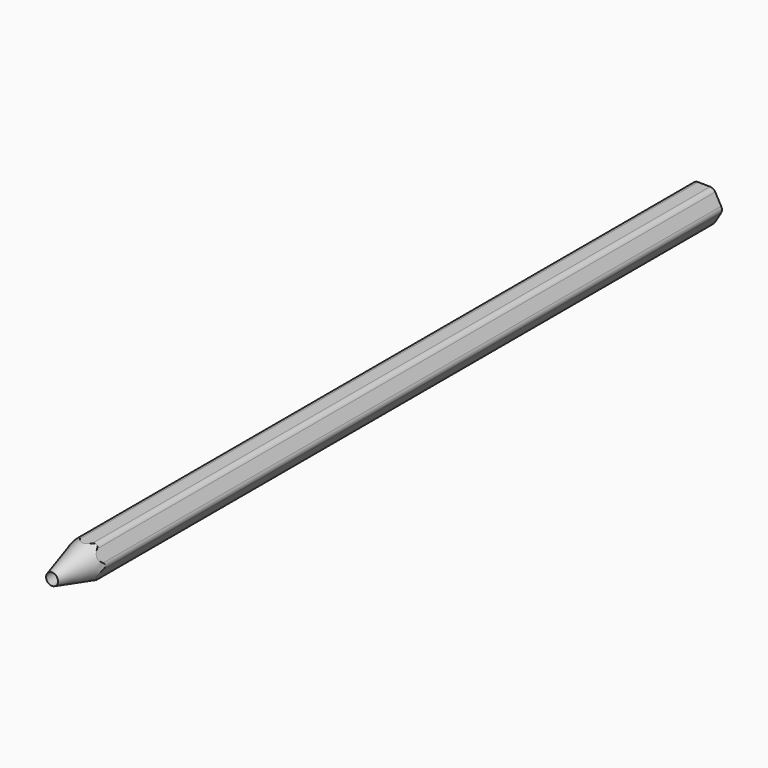
from build123d import *

# Parameters (mm, degrees)
F0_R        = 1.27
F1_DEPTH    = 88.9
F5_T1_DEPTH = 181.4661742094


# Not quite as in the source:
# - a fillet or chamfer that OpenCascade refuses, or shapes differently, is made with other operations: its cross-section is extruded or revolved along the edge and cut away or added


with BuildPart() as f1:
    # F0 (on Front) → F1 (new body, symmetric)
    with BuildSketch(Plane.XZ):
        Polygon((4.0324625191, -0.0515205351), (2.0608493518, 3.4664547138), (-1.9716131673, 3.5179752489), (-4.0324625191, 0.0515205351), (-2.0608493518, -3.4664547138), (1.9716131673, -3.5179752489), align=None)
        Circle(F0_R, mode=Mode.SUBTRACT)
    extrude(amount=F1_DEPTH, both=True)

    # F2 (on Top) → F4 (revolve, cut)
    with BuildSketch(Plane.XY):
        Polygon((0, -99.6820554137), (0, -88.9), (-4.0324625191, -74.2031688439), (-4.0324625191, -99.6820554137), align=None)
    revolve(axis=Axis((0, -76.0434828699, 0), (0, -1, 0)), mode=Mode.SUBTRACT)

    # F5: fillet of radius 1.27 on 6 edges, made by hand

    # F5_s2 → F5_t1 (cut)
    with BuildSketch(Plane.XZ.offset(-90.7330871047)):
        with BuildLine():
            ThreePointArc((2.4193244731, 2.8268228503), (1.960448821, 3.2975758517), (1.3276743483, 3.4758220838))
            Line((1.3276743483, 3.4758220838), (2.0608493518, 3.4664547138))
            Line((2.0608493518, 3.4664547138), (2.4193244731, 2.8268228503))
        make_face()
        with BuildLine():
            ThreePointArc((-1.2384381638, 3.5086078789), (-1.875560048, 3.3465864076), (-2.3463130494, 2.8877107555))
            Line((-2.3463130494, 2.8877107555), (-1.9716131673, 3.5179752489))
            Line((-1.9716131673, 3.5179752489), (-1.2384381638, 3.5086078789))
        make_face()
        with BuildLine():
            ThreePointArc((-3.6739873978, -0.5881113283), (-3.836008869, 0.0490105559), (-3.6577626369, 0.6817850286))
            Line((-3.6577626369, 0.6817850286), (-4.0324625191, 0.0515205351))
            Line((-4.0324625191, 0.0515205351), (-3.6739873978, -0.5881113283))
        make_face()
        with BuildLine():
            ThreePointArc((-1.3276743483, -3.4758220838), (-1.960448821, -3.2975758517), (-2.4193244731, -2.8268228503))
            Line((-2.4193244731, -2.8268228503), (-2.0608493518, -3.4664547138))
            Line((-2.0608493518, -3.4664547138), (-1.3276743483, -3.4758220838))
        make_face()
        with BuildLine():
            ThreePointArc((2.3463130494, -2.8877107555), (1.875560048, -3.3465864076), (1.2384381638, -3.5086078789))
            Line((1.2384381638, -3.5086078789), (1.9716131673, -3.5179752489))
            Line((1.9716131673, -3.5179752489), (2.3463130494, -2.8877107555))
        make_face()
        with BuildLine():
            ThreePointArc((3.6577626369, -0.6817850286), (3.836008869, -0.0490105559), (3.6739873978, 0.5881113283))
            Line((3.6739873978, 0.5881113283), (4.0324625191, -0.0515205351))
            Line((4.0324625191, -0.0515205351), (3.6577626369, -0.6817850286))
        make_face()
    extrude(amount=F5_T1_DEPTH, mode=Mode.SUBTRACT)


solid = f1.part
